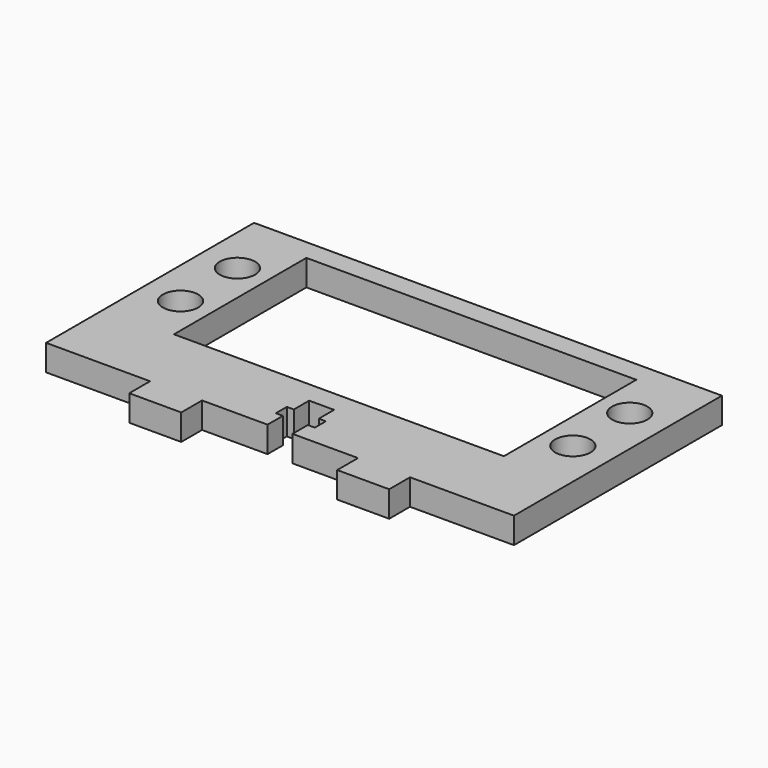
from build123d import *

# Parameters (mm, degrees)
F0_R     = 2.159
F0_W     = 40.3
F0_H     = 20.2184
F1_DEPTH = 3.175


# Not quite as in the source:
# - a length typed as a fraction of an inch, garbled in the dataset ("3 / 203.2 mm" for 3/8 in), is restored


with BuildPart() as f1:
    # F0 (on Top) → F1 (new body)
    with BuildSketch(Plane.XY):
        Polygon((28.575, -19.1008), (28.575, 12.6492), (-28.575, 12.6492), (-28.575, -19.1008), (-15.875, -19.1008), (-15.875, -22.2758), (-9.525, -22.2758), (-9.525, -19.1008), (-1.524, -19.1008), (-1.524, -16.764), (-2.38125, -16.764), (-2.38125, -15.0876), (-1.524, -15.0876), (-1.524, -12.7508), (1.524, -12.7508), (1.524, -15.0876), (2.38125, -15.0876), (2.38125, -16.764), (1.524, -16.764), (1.524, -19.1008), (9.525, -19.1008), (9.525, -22.2758), (15.875, -22.2758), (15.875, -19.1008), align=None)
        with Locations((-23.96, -4.3434)):
            Circle(F0_R, mode=Mode.SUBTRACT)
        with Locations((-23.96, 4.3434)):
            Circle(F0_R, mode=Mode.SUBTRACT)
        Rectangle(F0_W, F0_H, mode=Mode.SUBTRACT)
        with Locations((23.96, -4.3434)):
            Circle(F0_R, mode=Mode.SUBTRACT)
        with Locations((23.96, 4.3434)):
            Circle(F0_R, mode=Mode.SUBTRACT)
    extrude(amount=F1_DEPTH)


solid = f1.part
